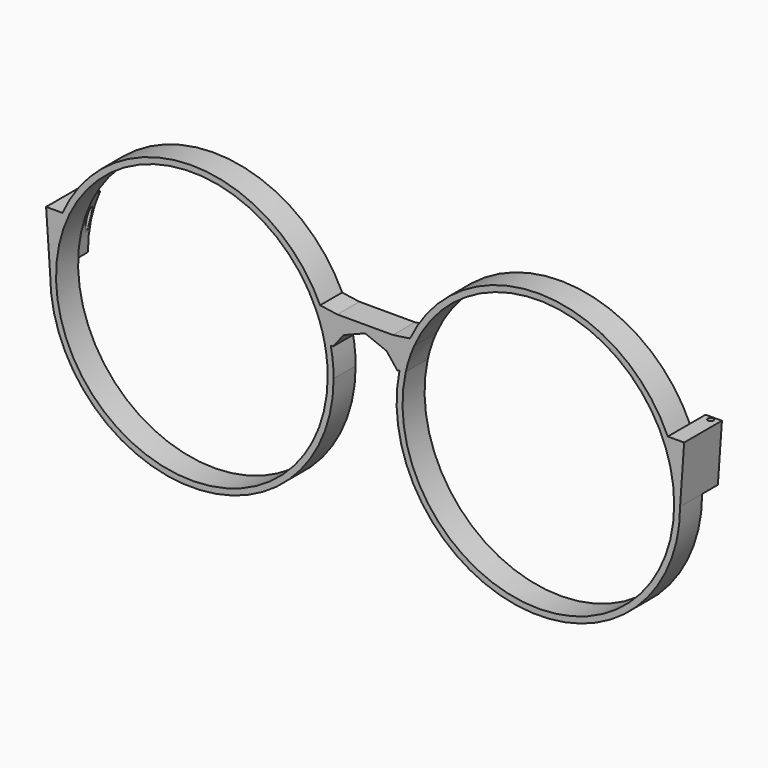
from build123d import *

# Parameters (mm, degrees)
F1_DEPTH = 7
F2_DEPTH = 5
F3_R     = 0.7
F4_DEPTH = 36.001


# Not quite as in the source:
# - a feature names something its author has since deleted; it is built from what else it names


with BuildPart() as f1:
    # F0 (on Front) → F1 (new body)
    with BuildSketch(Plane.XZ):
        with BuildLine():
            ThreePointArc((76.8747497611, 14.6714289741), (44.3508342177, 35.9982904504), (11.4174388077, 15.3093666149))
            Line((11.4174388077, 15.3093666149), (12.4627336019, 13.9875240173))
            ThreePointArc((12.4627336019, 13.9875240173), (51.1489268169, 33.7511902807), (78.5, 0))
            ThreePointArc((78.5, 0), (40.255323539, -34.2961717718), (10.312904452, 7.4451053411))
            Line((10.312904452, 7.4451053411), (8.7300367759, 7.2131611772))
            ThreePointArc((8.7300367759, 7.2131611772), (40.3749949013, -35.8170258122), (80, 0))
            ThreePointArc((80, 0), (79.2100198197, 7.5003002806), (76.8747497611, 14.6714289741))
        make_face()
        with BuildLine():
            ThreePointArc((-10.312904452, 7.4451053411), (-9.7038282282, 3.744676461), (-9.5, 0))
            ThreePointArc((-9.5, 0), (-77.7511902807, -7.1489268169), (-12.4627336019, 13.9875240173))
            Line((-12.4627336019, 13.9875240173), (-11.4174388077, 15.3093666149))
            ThreePointArc((-11.4174388077, 15.3093666149), (-44.3508342177, 35.9982904504), (-76.8747497611, 14.6714289741))
            ThreePointArc((-76.8747497611, 14.6714289741), (-79.2100198197, 7.5003002806), (-80, 0))
            ThreePointArc((-80, 0), (-44, -36), (-8, 0))
            ThreePointArc((-8, 0), (-8.1829741878, 3.6250050987), (-8.7300367759, 7.2131611772))
            Line((-8.7300367759, 7.2131611772), (-10.312904452, 7.4451053411))
        make_face()
        with BuildLine():
            ThreePointArc((-12.4627336019, 13.9875240173), (-11.2241680754, 10.7700901411), (-10.312904452, 7.4451053411))
            Line((-10.312904452, 7.4451053411), (-8.7300367759, 7.2131611772))
            ThreePointArc((-8.7300367759, 7.2131611772), (-9.8330802816, 11.3411461924), (-11.4174388077, 15.3093666149))
            Line((-11.4174388077, 15.3093666149), (-12.4627336019, 13.9875240173))
        make_face()
        with BuildLine():
            ThreePointArc((-11.4174388077, 15.3093666149), (-9.8330802816, 11.3411461924), (-8.7300367759, 7.2131611772))
            Line((-8.7300367759, 7.2131611772), (-8.1688707932, 7.1309311988))
            Line((-8.1688707932, 7.1309311988), (-5.43964638, 10.5822112661))
            Line((-5.43964638, 10.5822112661), (-7.0639303873, 14.6714289741))
            Line((-7.0639303873, 14.6714289741), (-11.4174388077, 15.3093666149))
        make_face()
        Polygon((0, 14.6714289741), (-7.0639303873, 14.6714289741), (-5.43964638, 10.5822112661), (0, 12.7429009753), (5.43964638, 10.5822112661), (7.0639303873, 14.6714289741), align=None)
        with BuildLine():
            Line((11.4174388077, 15.3093666149), (7.0639303873, 14.6714289741))
            Line((7.0639303873, 14.6714289741), (5.43964638, 10.5822112661))
            Line((5.43964638, 10.5822112661), (8.1688707932, 7.1309311988))
            Line((8.1688707932, 7.1309311988), (8.7300367759, 7.2131611772))
            ThreePointArc((8.7300367759, 7.2131611772), (9.8330802816, 11.3411461924), (11.4174388077, 15.3093666149))
        make_face()
        with BuildLine():
            Line((12.4627336019, 13.9875240173), (11.4174388077, 15.3093666149))
            ThreePointArc((11.4174388077, 15.3093666149), (9.8330802816, 11.3411461924), (8.7300367759, 7.2131611772))
            Line((8.7300367759, 7.2131611772), (10.312904452, 7.4451053411))
            ThreePointArc((10.312904452, 7.4451053411), (11.2241680754, 10.7700901411), (12.4627336019, 13.9875240173))
        make_face()
        with BuildLine():
            Line((81.0259262548, 14.6714289741), (76.8747497611, 14.6714289741))
            ThreePointArc((76.8747497611, 14.6714289741), (79.2100198197, 7.5003002806), (80, 0))
            Line((80, 0), (81.0259262548, 14.6714289741))
        make_face()
        with BuildLine():
            ThreePointArc((-80, 0), (-79.2100198197, 7.5003002806), (-76.8747497611, 14.6714289741))
            Line((-76.8747497611, 14.6714289741), (-81.0259262548, 14.6714289741))
            Line((-81.0259262548, 14.6714289741), (-80, 0))
        make_face()
    extrude(amount=F1_DEPTH)

    # F0 (on Front) → F2 (join)
    with BuildSketch(Plane.XZ):
        with BuildLine():
            ThreePointArc((-80, 0), (-79.2100198197, 7.5003002806), (-76.8747497611, 14.6714289741))
            Line((-76.8747497611, 14.6714289741), (-81.0259262548, 14.6714289741))
            Line((-81.0259262548, 14.6714289741), (-80, 0))
        make_face()
        with BuildLine():
            Line((81.0259262548, 14.6714289741), (76.8747497611, 14.6714289741))
            ThreePointArc((76.8747497611, 14.6714289741), (79.2100198197, 7.5003002806), (80, 0))
            Line((80, 0), (81.0259262548, 14.6714289741))
        make_face()
    extrude(amount=-F2_DEPTH)

    # F3 (on Top) → F4 (cut, through all)
    with BuildSketch(Plane.XY):
        with Locations((-78.950338008, 4)):
            Circle(F3_R)
        with Locations((78.950338008, 4)):
            Circle(F3_R)
    extrude(amount=F4_DEPTH, mode=Mode.SUBTRACT)


solid = f1.part
